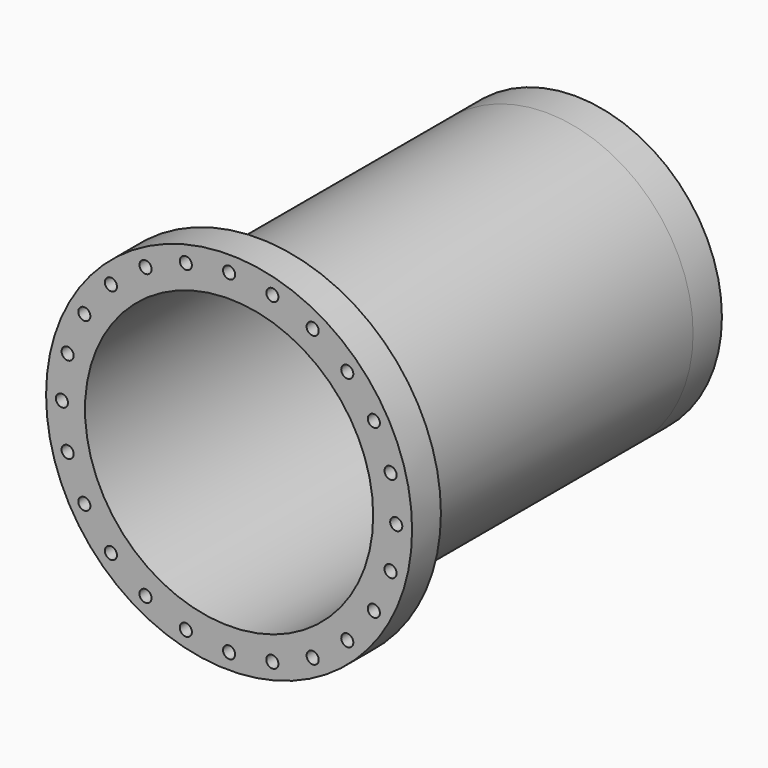
from build123d import *

# Parameters (mm, degrees)
F0_R      = 102
F0_R_2    = 100
F1_DEPTH  = 250
F2_R      = 127
F2_R_2    = 102
F2_R_3    = 100
F3_DEPTH  = 25
F4_R      = 102
F4_R_2    = 100
F5_DEPTH  = 25
F7_D      = 8.4
F8_R      = 50
F9_DEPTH  = 300.001
F10_D     = 8.4
F10_DEPTH = 9
F10_TIP   = 2.5236145999


with BuildPart() as f1:
    # F0 (on Front) → F1 (new body)
    with BuildSketch(Plane.XZ):
        Circle(F0_R)
        Circle(F0_R_2, mode=Mode.SUBTRACT)
    extrude(amount=F1_DEPTH)

    # F2 (on face) → F3 (join)
    with BuildSketch(Plane.XZ.offset(250)):
        Circle(F2_R)
        Circle(F2_R_2, mode=Mode.SUBTRACT)
        Circle(F2_R_2)
        Circle(F2_R_3, mode=Mode.SUBTRACT)
    extrude(amount=F3_DEPTH)

    # F4 (on face) → F5 (join)
    with BuildSketch(Plane(origin=(0, 0, 0), x_dir=(-1, 0, 0), z_dir=(0, 1, 0))):
        Circle(F4_R)
        Circle(F4_R_2, mode=Mode.SUBTRACT)
        Circle(F4_R_2)
    extrude(amount=F5_DEPTH)

    # F7 (through all)
    with Locations(Plane.XZ.offset(275)):
        with Locations((0, 116), (30.0230092319, 112.0473958495), (58, 100.458946839), (82.0243866176, 82.0243866176), (100.458946839, 58), (112.0473958495, 30.0230092319), (116, 0), (112.0473958495, -30.0230092319), (100.458946839, -58), (82.0243866176, -82.0243866176), (58, -100.458946839), (30.0230092319, -112.0473958495), (0, -116), (-30.0230092319, -112.0473958495), (-58, -100.458946839), (-82.0243866176, -82.0243866176), (-100.458946839, -58), (-112.0473958495, -30.0230092319), (-116, 0), (-112.0473958495, 30.0230092319), (-100.458946839, 58), (-82.0243866176, 82.0243866176), (-58, 100.458946839), (-30.0230092319, 112.0473958495)):
            Hole(F7_D / 2)

    # F8 (on face) → F9 (cut, through all)
    with BuildSketch(Plane(origin=(0, 25, 0), x_dir=(-1, 0, 0), z_dir=(0, 1, 0))):
        with Locations((5, 22.5)):
            Circle(F8_R)
    extrude(amount=-F9_DEPTH, mode=Mode.SUBTRACT)

    # F10
    with Locations(Plane(origin=(0, 25, 0), x_dir=(-1, 0, 0), z_dir=(0, 1, 0))):
        with Locations((5, 87.5), (-19.8744231037, -37.5521696132), (-40.9619407771, -23.4619407771), (-55.0521696132, -2.3744231037), (-60, 22.5), (-55.0521696132, 47.3744231037), (-40.9619407771, 68.4619407771), (-19.8744231037, 82.5521696132), (29.8744231037, 82.5521696132), (50.9619407771, 68.4619407771), (65.0521696132, 47.3744231037), (70, 22.5), (65.0521696132, -2.3744231037), (50.9619407771, -23.4619407771), (29.8744231037, -37.5521696132), (5, -42.5)):
            Hole(F10_D / 2, depth=F10_DEPTH)
            with Locations((0, 0, -(F10_DEPTH + F10_TIP / 2))):  # 118° drill point
                Cone(0, F10_D / 2, F10_TIP, mode=Mode.SUBTRACT)


solid = f1.part
